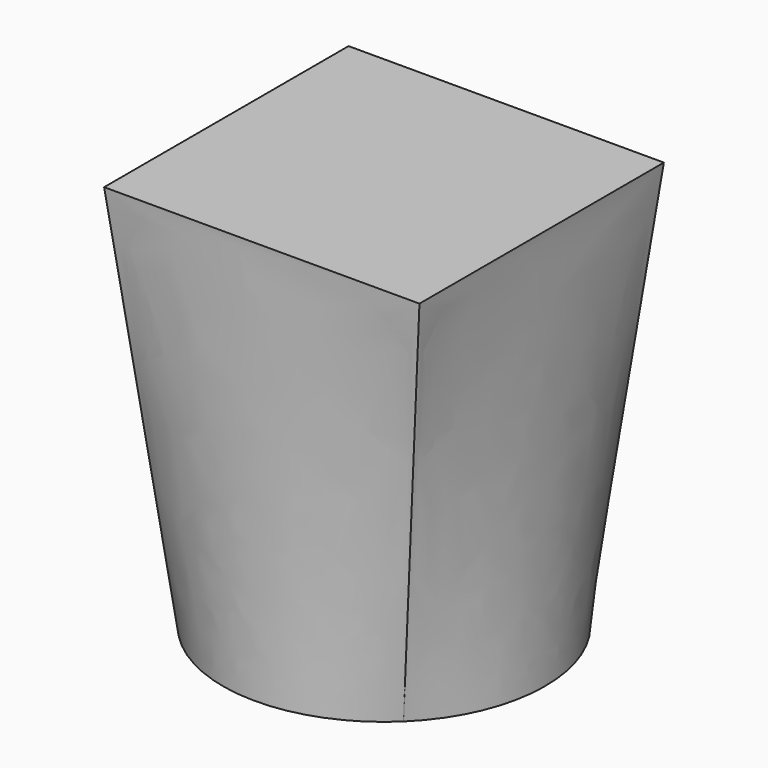
from build123d import *

# Parameters (mm, degrees)
F2_W = 60.4102350771
F2_H = 58.5308037698


# Not quite as in the source:
# - the arcs of a loft's sections are written as splines that run evenly, so that the points pair up as in the source's solid


with BuildPart() as f3:
    # F2 (on offset) → F3 section 0
    with BuildSketch(Plane.XY.offset(76.2)):
        Rectangle(F2_W, F2_H)
    # F1 (on Top) → F3 section 1
    with BuildSketch(Plane.XY):
        with BuildLine():
            add(Edge.make_bspline(
                [(22.1707526983, 21.4809952975), (20.7648248438, 22.9320676684), (19.2160171333, 24.2446357752), (15.892010091, 26.5424507837), (14.1168929518, 27.5276408675), (10.4084743028, 29.1328224007), (8.4752644909, 29.7527741589), (4.5249466842, 30.6036359906), (2.5079363687, 30.8345250249), (-1.5324720978, 30.8983690121), (-3.5557703417, 30.7313223864), (-7.5309988365, 30.0056950405), (-9.482830792, 29.4471322629), (-13.2401135133, 27.9599190359), (-15.0454713729, 27.0313053607), (-18.440418053, 24.8396590228), (-20.0299229267, 23.5766805529), (-21.4809952975, 22.1707526983)],
                knots=[0, 0, 0, 0, 0.125, 0.125, 0.25, 0.25, 0.375, 0.375, 0.5, 0.5, 0.625, 0.625, 0.75, 0.75, 0.875, 0.875, 1, 1, 1, 1], degree=3))
            add(Edge.make_bspline(
                [(-21.4809952975, 22.1707526983), (-22.9320676684, 20.7648248438), (-24.2446357752, 19.2160171333), (-26.5424507837, 15.892010091), (-27.5276408675, 14.1168929518), (-29.1328224007, 10.4084743028), (-29.7527741589, 8.4752644909), (-30.6036359906, 4.5249466842), (-30.8345250249, 2.5079363687), (-30.8983690121, -1.5324720978), (-30.7313223864, -3.5557703417), (-30.0056950405, -7.5309988365), (-29.4471322629, -9.482830792), (-27.9599190359, -13.2401135133), (-27.0313053607, -15.0454713729), (-24.8396590228, -18.440418053), (-23.5766805529, -20.0299229267), (-22.1707526983, -21.4809952975)],
                knots=[0, 0, 0, 0, 0.125, 0.125, 0.25, 0.25, 0.375, 0.375, 0.5, 0.5, 0.625, 0.625, 0.75, 0.75, 0.875, 0.875, 1, 1, 1, 1], degree=3))
            add(Edge.make_bspline(
                [(-22.1707526983, -21.4809952975), (-20.7648248438, -22.9320676684), (-19.2160171333, -24.2446357752), (-15.892010091, -26.5424507837), (-14.1168929518, -27.5276408675), (-10.4084743028, -29.1328224007), (-8.4752644909, -29.7527741589), (-4.5249466842, -30.6036359906), (-2.5079363687, -30.8345250249), (1.5324720978, -30.8983690121), (3.5557703417, -30.7313223864), (7.5309988365, -30.0056950405), (9.482830792, -29.4471322629), (13.2401135133, -27.9599190359), (15.0454713729, -27.0313053607), (18.440418053, -24.8396590228), (20.0299229267, -23.5766805529), (21.4809952975, -22.1707526983)],
                knots=[0, 0, 0, 0, 0.125, 0.125, 0.25, 0.25, 0.375, 0.375, 0.5, 0.5, 0.625, 0.625, 0.75, 0.75, 0.875, 0.875, 1, 1, 1, 1], degree=3))
            add(Edge.make_bspline(
                [(21.4809952975, -22.1707526983), (22.9320676684, -20.7648248438), (24.2446357752, -19.2160171333), (26.5424507837, -15.892010091), (27.5276408675, -14.1168929518), (29.1328224007, -10.4084743028), (29.7527741589, -8.4752644909), (30.6036359906, -4.5249466842), (30.8345250249, -2.5079363687), (30.8983690121, 1.5324720978), (30.7313223864, 3.5557703417), (30.0056950405, 7.5309988365), (29.4471322629, 9.482830792), (27.9599190359, 13.2401135133), (27.0313053607, 15.0454713729), (24.8396590228, 18.440418053), (23.5766805529, 20.0299229267), (22.1707526983, 21.4809952975)],
                knots=[0, 0, 0, 0, 0.125, 0.125, 0.25, 0.25, 0.375, 0.375, 0.5, 0.5, 0.625, 0.625, 0.75, 0.75, 0.875, 0.875, 1, 1, 1, 1], degree=3))
        make_face()
    loft(ruled=True)


solid = f3.part
